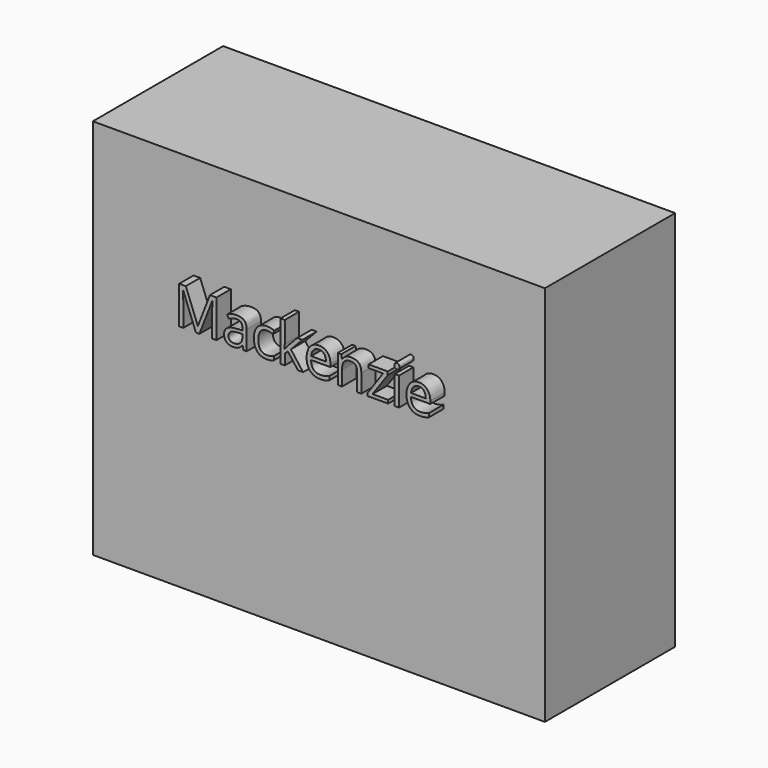
from build123d import *

# Parameters (mm, degrees)
F0_W         = 70.5273374915
F0_H         = 59.5630016178
F1_DEPTH     = 25.4
F2_TEXT_SIZE = 8.2196033974
F3_DEPTH     = 28.194


# Not quite as in the source:
# - Text() gives the source's letters only with a copy of the font that has no kerning and outlines rounded to 1/6400 em; it was checked with that copy


with BuildPart() as f1:
    # F0 (on Front) → F1 (new body)
    with BuildSketch(Plane.XZ):
        with Locations((2.2225007415, -2.5188336149)):
            Rectangle(F0_W, F0_H)
    extrude(amount=F1_DEPTH)

    # F2 (on Front) → F3 (join)
    with BuildSketch(Plane.XZ):
        with Locations((-18.1349124759, 5.32723777)):
            Text('Mackenzie', F2_TEXT_SIZE, font='Open Sans', text_align=(TextAlign.LEFT, TextAlign.BOTTOM))
    extrude(amount=F3_DEPTH)


solid = f1.part
